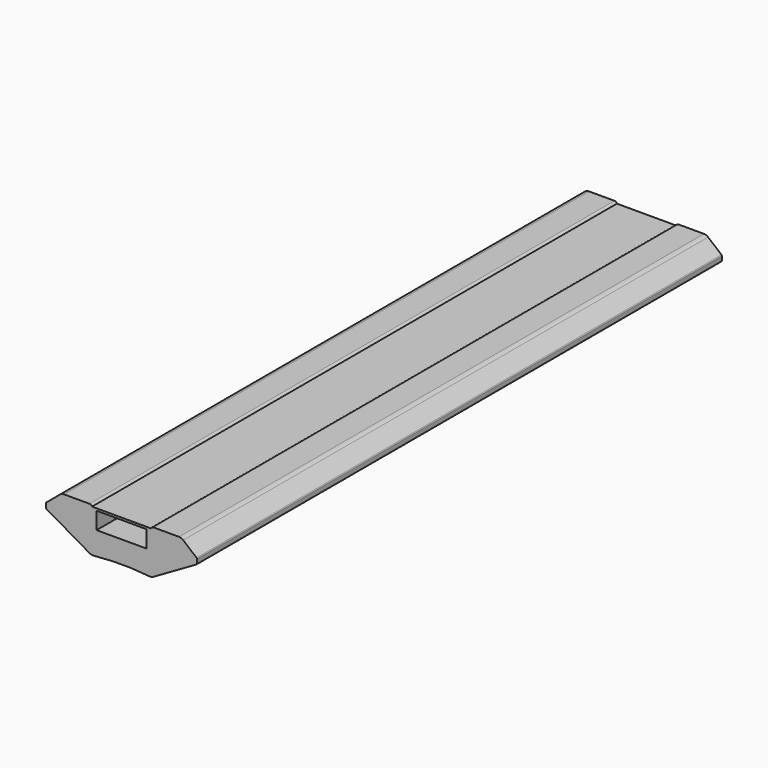
from build123d import *

# Parameters (mm, degrees)
F1_DEPTH    = 250
F2_R        = 5
F3_R        = 1
F4_W        = 38
F4_H        = 13
F5_DEPTH    = 500.001
F6_T1_DEPTH = 509.3674969976


# Not quite as in the source:
# - a fillet or chamfer that OpenCascade refuses, or shapes differently, is made with other operations: its cross-section is extruded or revolved along the edge and cut away or added


with BuildPart() as f1:
    # F0 (on Front) → F1 (new body, symmetric)
    with BuildSketch(Plane.XZ):
        with BuildLine():
            Line((22.5, 29.7386717319), (0, 29.7386717319))
            Line((0, 29.7386717319), (-22.5, 29.7386717319))
            Line((-22.5, 29.7386717319), (-22.5, 31.0386717319))
            Line((-22.5, 31.0386717319), (-45.5824640741, 31.0386717319))
            Line((-45.5824640741, 31.0386717319), (-57.5, 21.0386717319))
            Line((-57.5, 21.0386717319), (-57.5, 17.0386717319))
            Line((-57.5, 17.0386717319), (-22.8589838486, -2.9613282681))
            ThreePointArc((-22.8589838486, -2.9613282681), (0, -1.6507010523), (22.8589838486, -2.9613282681))
            Line((22.8589838486, -2.9613282681), (57.5, 17.0386717319))
            Line((57.5, 17.0386717319), (57.5, 21.0386717319))
            Line((57.5, 21.0386717319), (45.5824640741, 31.0386717319))
            Line((45.5824640741, 31.0386717319), (22.5, 31.0386717319))
            Line((22.5, 31.0386717319), (22.5, 29.7386717319))
        make_face()
    extrude(amount=F1_DEPTH, both=True)

    # F2
    f2_edges = [f1.edges().sort_by_distance(p)[0] for p in [
        (45.582464, 0, 31.038672),
        (22.858984, 0, -2.961328),
        (-45.582464, 0, 31.038672),
        (-22.858984, 0, -2.961328),
    ]]
    fillet(f2_edges, radius=F2_R)

    # F3
    f3_edges = [f1.edges().sort_by_distance(p)[0] for p in [
        (57.5, 0, 21.038672),
        (57.5, 0, 17.038672),
        (-57.5, 0, 21.038672),
        (-57.5, 0, 17.038672),
    ]]
    fillet(f3_edges, radius=F3_R)

    # F4 (on face) → F5 (cut, through all)
    with BuildSketch(Plane.XZ.offset(250)):
        with Locations((0, 21.5986846235)):
            Rectangle(F4_W, F4_H)
    extrude(amount=-F5_DEPTH, mode=Mode.SUBTRACT)

    # F6: fillet of radius 2 on 2 edges, made by hand

    # F6_s2 → F6_t1 (cut)
    with BuildSketch(Plane.XZ.offset(-254.6837484988)):
        with BuildLine():
            ThreePointArc((-22.5, 29.7386717319), (-23.2333239744, 30.6818394045), (-24.3734993995, 31.0386717319))
            Line((-24.3734993995, 31.0386717319), (-22.5, 31.0386717319))
            Line((-22.5, 31.0386717319), (-22.5, 29.7386717319))
        make_face()
        with BuildLine():
            ThreePointArc((24.3734993995, 31.0386717319), (23.2333239744, 30.6818394045), (22.5, 29.7386717319))
            Line((22.5, 29.7386717319), (22.5, 31.0386717319))
            Line((22.5, 31.0386717319), (24.3734993995, 31.0386717319))
        make_face()
    extrude(amount=F6_T1_DEPTH, mode=Mode.SUBTRACT)


solid = f1.part
